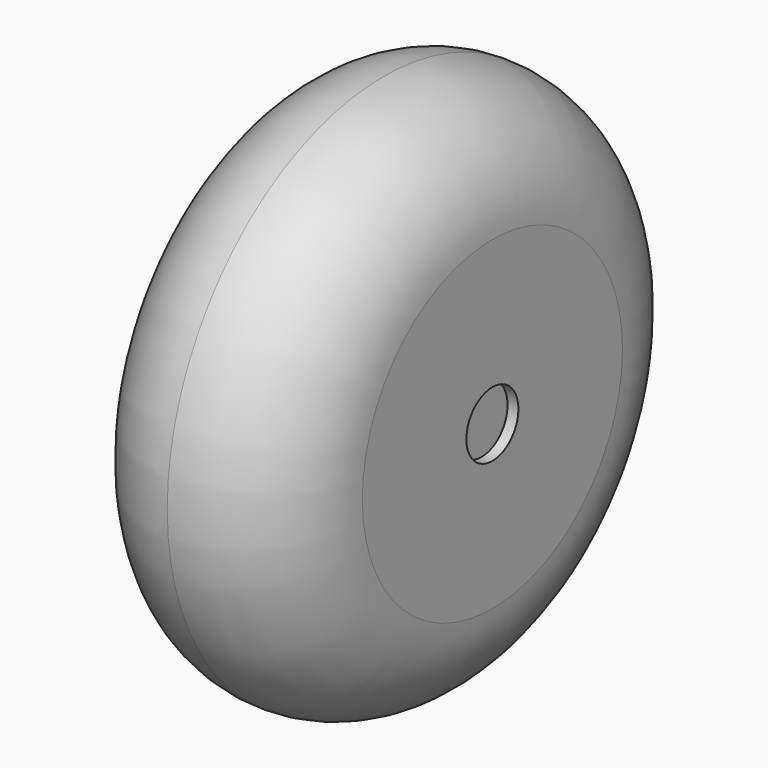
from build123d import *

# Parameters (mm, degrees)
F0_R     = 6.35
F1_DEPTH = 5.08
F2_R     = 2.53999
F3_R     = 0.762
F4_DEPTH = 0.254


# Not quite as in the source:
# - a fillet or chamfer is up to 0.001 mm smaller than in the source, because OpenCascade refuses the exact size


with BuildPart() as f1:
    # F0 (on Right) → F1 (new body)
    with BuildSketch(Plane.YZ):
        Circle(F0_R)
    extrude(amount=F1_DEPTH)

    # F2 (radius 2.54 in the source; OpenCascade refuses exactly that, so slightly less here)
    f2_edges = [f1.edges().sort_by_distance(p)[0] for p in [
        (5.08, -6.35, 0),
        (0, -6.35, 0),
    ]]
    fillet(f2_edges, radius=F2_R)

    # F3 (on face) → F4 (cut)
    with BuildSketch(Plane.YZ.offset(5.08)):
        Circle(F3_R)
    extrude(amount=-F4_DEPTH, mode=Mode.SUBTRACT)


solid = f1.part
